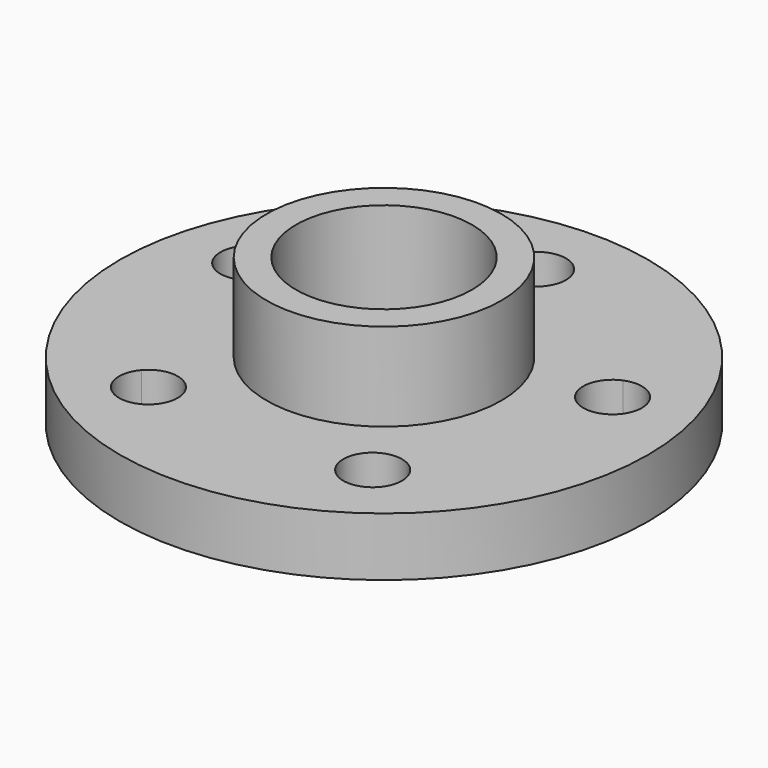
from build123d import *

# Parameters (mm, degrees)
F3_DEPTH = 10.001


with BuildPart() as f1:
    # F0 (on Front) → F1 (revolve)
    with BuildSketch(Plane.XZ):
        Polygon((20, 25), (15, 25), (15, 0), (45, 0), (45, 10), (20, 10), align=None)
    revolve(axis=Axis((0, 0, 17.8506122556), (0, 0, -1)))

    # F2 (on face) → F3 (cut, through all)
    with BuildSketch(Plane.XY.offset(10)):
        with BuildLine():
            ThreePointArc((29.0030388795, 14.6653924514), (26.1540541981, 8.4979673453), (32.0840527441, 5.1830068027))
            ThreePointArc((32.0840527441, 5.1830068027), (30.9093367796, 10.0430523172), (29.0030388795, 14.6653924514))
        make_face()
        with BuildLine():
            ThreePointArc((29.0030388795, 14.6653924514), (30.9093367796, 10.0430523172), (32.0840527441, 5.1830068027))
            ThreePointArc((32.0840527441, 5.1830068027), (34.8383048262, 6.9506082855), (35.9093367796, 10.0430523172))
            ThreePointArc((35.9093367796, 10.0430523172), (33.6903896827, 14.1982592615), (29.0030388795, 14.6653924514))
        make_face()
        with BuildLine():
            ThreePointArc((24.1030206995, -26.2930523172), (23.7953091225, -24.5660811664), (22.9100489572, -23.0516736221))
            ThreePointArc((22.9100489572, -23.0516736221), (19.1030206995, -26.2930523172), (14.84384994, -28.9121102474))
            ThreePointArc((14.84384994, -28.9121102474), (20.4639296242, -31.1042815675), (24.1030206995, -26.2930523172))
        make_face()
        with BuildLine():
            ThreePointArc((14.84384994, -28.9121102474), (19.1030206995, -26.2930523172), (22.9100489572, -23.0516736221))
            ThreePointArc((22.9100489572, -23.0516736221), (16.164094438, -22.2479673453), (14.84384994, -28.9121102474))
        make_face()
        with BuildLine():
            ThreePointArc((-4.9851851526, 32.1153846154), (0, 27.5), (4.9851851526, 32.1153846154))
            ThreePointArc((4.9851851526, 32.1153846154), (0, 32.5), (-4.9851851526, 32.1153846154))
        make_face()
        with BuildLine():
            ThreePointArc((-4.9851851526, 32.1153846154), (0, 32.5), (4.9851851526, 32.1153846154))
            ThreePointArc((4.9851851526, 32.1153846154), (4.9962949154, 32.3075496988), (5, 32.5))
            ThreePointArc((5, 32.5), (-0.1924503012, 37.4962949154), (-4.9851851526, 32.1153846154))
        make_face()
        with BuildLine():
            ThreePointArc((-22.9100489572, -23.0516736221), (-22.041946961, -30.3381372891), (-14.84384994, -28.9121102474))
            ThreePointArc((-14.84384994, -28.9121102474), (-19.1030206995, -26.2930523172), (-22.9100489572, -23.0516736221))
        make_face()
        with BuildLine():
            ThreePointArc((-22.9100489572, -23.0516736221), (-19.1030206995, -26.2930523172), (-14.84384994, -28.9121102474))
            ThreePointArc((-14.84384994, -28.9121102474), (-14.2917914492, -27.6539612419), (-14.1030206995, -26.2930523172))
            ThreePointArc((-14.1030206995, -26.2930523172), (-17.3760495487, -21.6007638942), (-22.9100489572, -23.0516736221))
        make_face()
        with BuildLine():
            ThreePointArc((-25.9093367796, 10.0430523172), (-26.7541298353, 12.8241052203), (-29.0030388795, 14.6653924514))
            ThreePointArc((-29.0030388795, 14.6653924514), (-30.9093367796, 10.0430523172), (-32.0840527441, 5.1830068027))
            ThreePointArc((-32.0840527441, 5.1830068027), (-27.8168927479, 6.1140842706), (-25.9093367796, 10.0430523172))
        make_face()
        with BuildLine():
            ThreePointArc((-32.0840527441, 5.1830068027), (-30.9093367796, 10.0430523172), (-29.0030388795, 14.6653924514))
            ThreePointArc((-29.0030388795, 14.6653924514), (-35.6646193611, 11.5881372891), (-32.0840527441, 5.1830068027))
        make_face()
    extrude(amount=-F3_DEPTH, mode=Mode.SUBTRACT)


solid = f1.part
